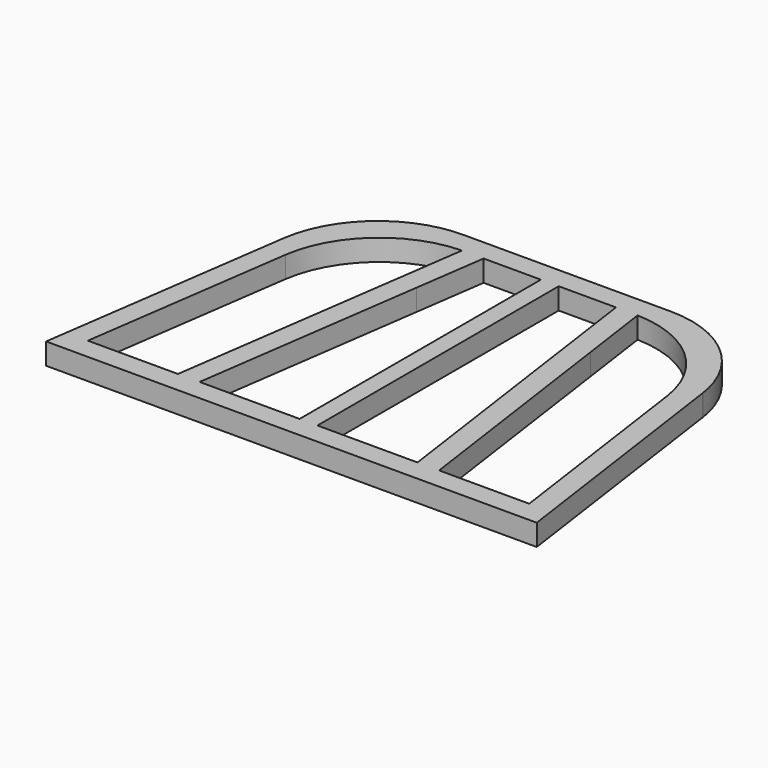
from build123d import *

# Parameters (mm, degrees)
F1_DEPTH    = 12
F2_T1_DEPTH = 12
F3_R        = 60


# Not quite as in the source:
# - a fillet or chamfer that OpenCascade refuses, or shapes differently, is made with other operations: its cross-section is extruded or revolved along the edge and cut away or added


with BuildPart() as f1:
    # F0 (on Top) → F1 (new body)
    with BuildSketch(Plane.XY):
        Polygon((132.5, 193), (132.5, 181), (137.5, 181), (142.5, 181), (142.5, 193), (137.5, 193), align=None)
        Polygon((27.3656716418, 193), (25.6641791045, 181), (37.7842070275, 181), (39.4856995648, 193), align=None)
        Polygon((25.6641791045, 181), (19.9925373134, 141), (32.1125652364, 141), (37.7842070275, 181), align=None)
        Polygon((19.9925373134, 141), (18.2910447761, 129), (30.4110726991, 129), (32.1125652364, 141), align=None)
        Polygon((237.2157929725, 181), (242.8874347636, 141), (255.0074626866, 141), (249.3358208955, 181), align=None)
        Polygon((235.5143004352, 193), (237.2157929725, 181), (249.3358208955, 181), (247.6343283582, 193), align=None)
        Polygon((242.8874347636, 141), (244.5889273009, 129), (256.7089552239, 129), (255.0074626866, 141), align=None)
        Polygon((244.5889273009, 129), (251.6784795397, 79), (263.7985074627, 79), (256.7089552239, 129), align=None)
        Polygon((251.6784795397, 79), (253.379972077, 67), (265.5, 67), (263.7985074627, 79), align=None)
        Polygon((132.5, 79), (132.5, 67), (137.5, 67), (142.5, 67), (142.5, 79), (137.5, 79), align=None)
        Polygon((253.379972077, 67), (261.1784795397, 12), (273.2985074627, 12), (265.5, 67), align=None)
        Polygon((261.1784795397, 12), (262.879972077, 0), (275, 0), (273.2985074627, 12), align=None)
        Polygon((13.8215204603, 12), (12.120027923, 0), (62.6201442689, 0), (64.3216368062, 12), align=None)
        Polygon((1.7014925373, 12), (0, 0), (12.120027923, 0), (13.8215204603, 12), align=None)
        Polygon((9.5, 67), (1.7014925373, 12), (13.8215204603, 12), (21.620027923, 67), align=None)
        Polygon((11.2014925373, 79), (9.5, 67), (21.620027923, 67), (23.3215204603, 79), align=None)
        Polygon((18.2910447761, 129), (11.2014925373, 79), (23.3215204603, 79), (30.4110726991, 129), align=None)
        Polygon((132.5, 141), (132.5, 129), (137.5, 129), (142.5, 129), (142.5, 141), (137.5, 141), align=None)
        Polygon((72.1201442689, 67), (64.3216368062, 12), (76.4416647292, 12), (84.2401721919, 67), align=None)
        Polygon((80.911189045, 129), (73.8216368062, 79), (85.9416647292, 79), (93.031216968, 129), align=None)
        Polygon((88.2843233734, 181), (82.6126815823, 141), (94.7327095053, 141), (100.4043512964, 181), align=None)
        Polygon((39.4856995648, 193), (37.7842070275, 181), (88.2843233734, 181), (89.9858159107, 193), align=None)
        Polygon((102.1058438337, 193), (100.4043512964, 181), (132.5, 181), (132.5, 193), align=None)
        Polygon((142.5, 193), (142.5, 181), (174.5956487036, 181), (172.8941561663, 193), align=None)
        Polygon((185.0141840893, 193), (186.7156766266, 181), (237.2157929725, 181), (235.5143004352, 193), align=None)
        Polygon((172.8941561663, 193), (174.5956487036, 181), (186.7156766266, 181), (185.0141840893, 193), align=None)
        Polygon((174.5956487036, 181), (180.2672904947, 141), (192.3873184177, 141), (186.7156766266, 181), align=None)
        Polygon((180.2672904947, 141), (181.968783032, 129), (194.088810955, 129), (192.3873184177, 141), align=None)
        Polygon((181.968783032, 129), (189.0583352708, 79), (201.1783631938, 79), (194.088810955, 129), align=None)
        Polygon((189.0583352708, 79), (190.7598278081, 67), (202.8798557311, 67), (201.1783631938, 79), align=None)
        Polygon((190.7598278081, 67), (198.5583352708, 12), (210.6783631938, 12), (202.8798557311, 67), align=None)
        Polygon((210.6783631938, 12), (212.3798557311, 0), (262.879972077, 0), (261.1784795397, 12), align=None)
        Polygon((198.5583352708, 12), (200.2598278081, 0), (212.3798557311, 0), (210.6783631938, 12), align=None)
        Polygon((142.5, 12), (142.5, 0), (200.2598278081, 0), (198.5583352708, 12), align=None)
        Polygon((132.5, 12), (132.5, 0), (142.5, 0), (142.5, 12), (137.5, 12), align=None)
        Polygon((76.4416647292, 12), (74.7401721919, 0), (132.5, 0), (132.5, 12), align=None)
        Polygon((64.3216368062, 12), (62.6201442689, 0), (74.7401721919, 0), (76.4416647292, 12), align=None)
        Polygon((132.5, 67), (132.5, 12), (137.5, 12), (142.5, 12), (142.5, 67), (137.5, 67), align=None)
        Polygon((132.5, 129), (132.5, 79), (137.5, 79), (142.5, 79), (142.5, 129), (137.5, 129), align=None)
        Polygon((132.5, 181), (132.5, 141), (137.5, 141), (142.5, 141), (142.5, 181), (137.5, 181), align=None)
        Polygon((89.9858159107, 193), (88.2843233734, 181), (100.4043512964, 181), (102.1058438337, 193), align=None)
        Polygon((82.6126815823, 141), (80.911189045, 129), (93.031216968, 129), (94.7327095053, 141), align=None)
        Polygon((73.8216368062, 79), (72.1201442689, 67), (84.2401721919, 67), (85.9416647292, 79), align=None)
    extrude(amount=F1_DEPTH)

    # F2: fillet of radius 60 on 2 edges, made by hand

    # F2_s2 → F2_t1 (join)
    with BuildSketch(Plane.XY):
        with BuildLine():
            ThreePointArc((186.7156872707, 181.0003998584), (225.0552814168, 165.8005010735), (244.5264534747, 129.4434541493))
            Line((244.5264534747, 129.4434541493), (250.4671955698, 130.2857981777))
            ThreePointArc((250.4671955698, 130.2857981777), (246.8116672993, 156.0640430257), (243.1565350676, 181.8423440284))
            Line((243.1565350676, 181.8423440284), (237.2157929725, 187.0001633397))
            ThreePointArc((237.2157929725, 187.0001633397), (211.9657401216, 187.0001633397), (186.8753527454, 186.9984384577))
            Line((186.8753527454, 186.9984384577), (186.7156872707, 181.0003998584))
        make_face()
        with BuildLine():
            ThreePointArc((30.4735465253, 129.4434541493), (49.9447185832, 165.8005010735), (88.2843127293, 181.0003998584))
            Line((88.2843127293, 181.0003998584), (88.1246472546, 186.9984384577))
            ThreePointArc((88.1246472546, 186.9984384577), (63.0342598784, 187.0001633397), (37.7842070275, 187.0001633397))
            Line((37.7842070275, 187.0001633397), (31.8434649324, 181.8423440284))
            ThreePointArc((31.8434649324, 181.8423440284), (28.1883327007, 156.0640430257), (24.5328044302, 130.2857981777))
            Line((24.5328044302, 130.2857981777), (30.4735465253, 129.4434541493))
        make_face()
    extrude(amount=F2_T1_DEPTH)

    # F3
    f3_edges = [f1.edges().sort_by_distance(p)[0] for p in [
        (27.365672, 193, 6),
        (247.634328, 193, 6),
    ]]
    fillet(f3_edges, radius=F3_R)


solid = f1.part
